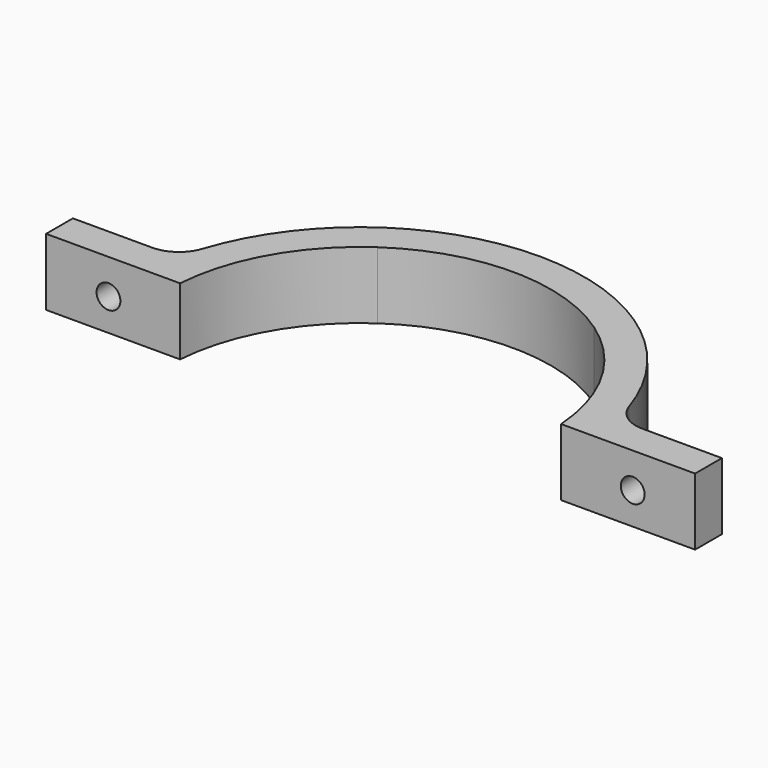
from build123d import *

# Parameters (mm, degrees)
F1_DEPTH = 10
F4_DEPTH = 10.001
F6_D     = 3.556
F7_R     = 5


# Not quite as in the source:
# - a feature of the source that left no trace in its solid (it failed there, or was rolled back) is left out
# - a feature names something its author has since deleted; it is built from what else it names


with BuildPart() as f1:
    # F0 (on Top) → F1 (new body)
    with BuildSketch(Plane.XY):
        with BuildLine():
            ThreePointArc((16.1705551086, 23.468343518), (24.7491207645, 14.1326225939), (28.4297379517, 2))
            Line((28.4297379517, 2), (28.4297379517, 7))
            Line((28.4297379517, 7), (32.7604945018, 7))
            ThreePointArc((32.7604945018, 7), (26.8945535829, 19.9733068763), (16.1705551086, 29.3387652685))
            Line((16.1705551086, 29.3387652685), (16.1705551086, 23.468343518))
        make_face()
        with BuildLine():
            ThreePointArc((-16.1705551086, 23.468343518), (0, 28.5), (16.1705551086, 23.468343518))
            Line((16.1705551086, 23.468343518), (16.1705551086, 29.3387652685))
            Line((16.1705551086, 29.3387652685), (-16.1705551086, 29.3387652685))
            Line((-16.1705551086, 29.3387652685), (-16.1705551086, 23.468343518))
        make_face()
        with BuildLine():
            ThreePointArc((-28.4297379517, 2), (-24.7491207645, 14.1326225939), (-16.1705551086, 23.468343518))
            Line((-16.1705551086, 23.468343518), (-16.1705551086, 29.3387652685))
            ThreePointArc((-16.1705551086, 29.3387652685), (-26.8945535829, 19.9733068763), (-32.7604945018, 7))
            Line((-32.7604945018, 7), (-28.4297379517, 7))
            Line((-28.4297379517, 7), (-28.4297379517, 2))
        make_face()
        with BuildLine():
            Line((-48.4297379517, 2), (-33.4402452144, 2))
            ThreePointArc((-33.4402452144, 2), (-33.1946454228, 4.5128167765), (-32.7604945018, 7))
            Line((-32.7604945018, 7), (-48.4297379517, 7))
            Line((-48.4297379517, 7), (-48.4297379517, 2))
        make_face()
        with BuildLine():
            Line((-33.4402452144, 2), (-28.4297379517, 2))
            Line((-28.4297379517, 2), (-28.4297379517, 7))
            Line((-28.4297379517, 7), (-32.7604945018, 7))
            ThreePointArc((-32.7604945018, 7), (-33.1946454228, 4.5128167765), (-33.4402452144, 2))
        make_face()
        with BuildLine():
            Line((28.4297379517, 7), (28.4297379517, 2))
            Line((28.4297379517, 2), (33.4402452144, 2))
            ThreePointArc((33.4402452144, 2), (33.1946454228, 4.5128167765), (32.7604945018, 7))
            Line((32.7604945018, 7), (28.4297379517, 7))
        make_face()
        with BuildLine():
            ThreePointArc((32.7604945018, 7), (33.1946454228, 4.5128167765), (33.4402452144, 2))
            Line((33.4402452144, 2), (48.4297379517, 2))
            Line((48.4297379517, 2), (48.4297379517, 7))
            Line((48.4297379517, 7), (32.7604945018, 7))
        make_face()
        with BuildLine():
            Line((-16.1705551086, 29.3387652685), (16.1705551086, 29.3387652685))
            ThreePointArc((16.1705551086, 29.3387652685), (8.3486935036, 32.4430164563), (1.811e-07, 33.5))
            ThreePointArc((1.811e-07, 33.5), (-8.3486933282, 32.4430165014), (-16.1705551086, 29.3387652685))
        make_face()
    extrude(amount=F1_DEPTH)

    # F0 (on Top) → F4 (cut, through all)
    with BuildSketch(Plane.XY):
        with BuildLine():
            Line((-16.1705551086, 23.468343518), (16.1705551086, 23.468343518))
            ThreePointArc((16.1705551086, 23.468343518), (0, 28.5), (-16.1705551086, 23.468343518))
        make_face()
    extrude(amount=F4_DEPTH, mode=Mode.SUBTRACT)

    # F6 (through all)
    with Locations(Plane.XZ.offset(-2)):
        with Locations((-39.116, 4.78035165), (39.116, 4.78035165)):
            Hole(F6_D / 2)

    # F7
    f7_edges = [f1.edges().sort_by_distance(p)[0] for p in [
        (-32.760495, 7, 5),
        (32.760495, 7, 5),
    ]]
    fillet(f7_edges, radius=F7_R)


solid = f1.part
